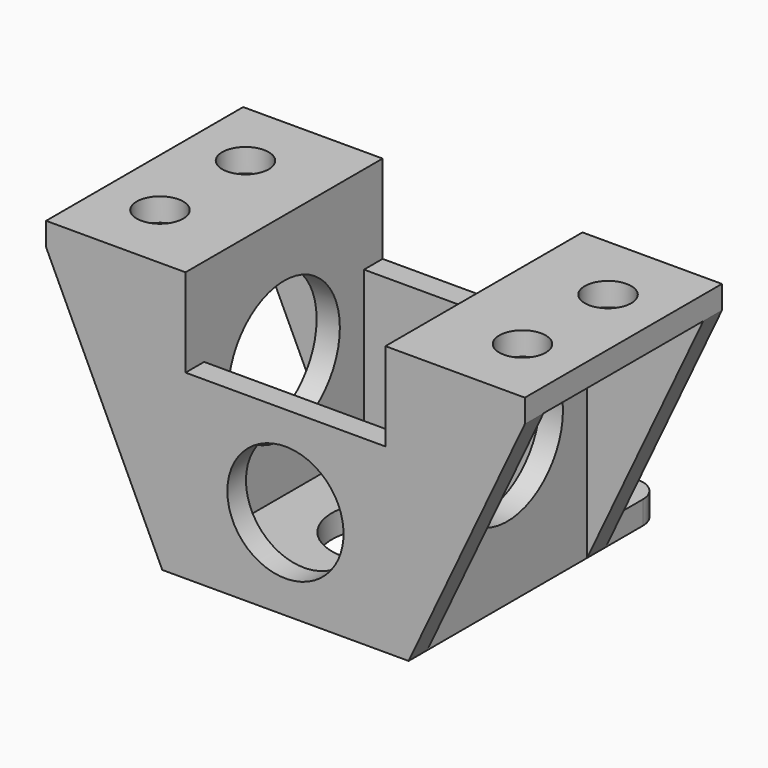
from build123d import *

# Parameters (mm, degrees)
F0_W      = 53
F0_H      = 53
F1_DEPTH  = 10
F2_W      = 43
F2_H      = 43
F3_DEPTH  = 5
F4_R      = 1.7
F5_DEPTH  = 25
F6_R      = 11.2
F7_DEPTH  = 25
F9_DEPTH  = 48
F10_DEPTH = 29
F11_R     = 15
F12_DEPTH = 53.001
F13_R     = 12.5
F14_DEPTH = 53.001
F15_W     = 5
F15_H     = 58
F16_DEPTH = 25
F17_SIZE2 = 53
F17_SIZE  = 25
F18_W     = 43
F18_H     = 5
F19_DEPTH = 25
F20_R     = 5
F21_DEPTH = 25
F22_W     = 15
F22_H     = 5
F23_DEPTH = 15
F24_R     = 5
F25_R     = 4
F26_DEPTH = 25


# Not quite as in the source:
# - a pattern or mirror of a feature is missing from the dataset's text; its kind, count and spacing are read off the source's solid


with BuildPart() as f1:
    # F0 (on Top) → F1 (new body)
    with BuildSketch(Plane.XY):
        Rectangle(F0_W, F0_H)
    extrude(amount=F1_DEPTH)

    # F2 (on face) → F3 (cut)
    with BuildSketch(Plane.XY.offset(10)):
        Rectangle(F2_W, F2_H)
    extrude(amount=-F3_DEPTH, mode=Mode.SUBTRACT)

    # F4 (on face) → F5 (cut)
    with BuildSketch(Plane(origin=(0, 0, 0), x_dir=(1, 0, 0), z_dir=(0, 0, -1))):
        with Locations((-16.5182938799, 16.5182938799)):
            Circle(F4_R)
        with Locations((16.0086180547, 16.5182938799)):
            Circle(F4_R)
        with Locations((16.0086180547, -16.0086180547)):
            Circle(F4_R)
        with Locations((-16.5182938799, -16.0086180547)):
            Circle(F4_R)
    extrude(amount=-F5_DEPTH, mode=Mode.SUBTRACT)

    # F6 (on face) → F7 (cut)
    with BuildSketch(Plane(origin=(0, 0, 0), x_dir=(1, 0, 0), z_dir=(0, 0, -1))):
        Circle(F6_R)
    extrude(amount=-F7_DEPTH, mode=Mode.SUBTRACT)

    # F8 (on face) → F9 (join)
    with BuildSketch(Plane.XY.offset(10)):
        Polygon((-21.5, -21.5), (-21.5, 21.5), (-21.5, 26.5), (-26.5, 26.5), (-26.5, -26.5), (-21.5, -26.5), align=None)
        Polygon((21.5, 26.5), (21.5, 21.5), (21.5, -21.5), (21.5, -26.5), (26.5, -26.5), (26.5, 26.5), align=None)
    extrude(amount=F9_DEPTH)

    # F10 (add): faces of the model
    f10_faces = [f1.faces().sort_by_distance(p)[0] for p in [
        (0, 24, 10),
        (0, -24, 10),
    ]]
    extrude(f10_faces, amount=F10_DEPTH)

    # F11 (on face) → F12 (cut, through all)
    with BuildSketch(Plane.YZ.offset(26.5)):
        with Locations((0, 30.6356716901)):
            Circle(F11_R)
    extrude(amount=-F12_DEPTH, mode=Mode.SUBTRACT)

    # F13 (on face) → F14 (cut, through all)
    with BuildSketch(Plane(origin=(0, 26.5, 0), x_dir=(-1, 0, 0), z_dir=(0, 1, 0))):
        with Locations((0, 19.5)):
            Circle(F13_R)
    extrude(amount=-F14_DEPTH, mode=Mode.SUBTRACT)

    # F15 (on face) → F16 (join)
    with BuildSketch(Plane(origin=(-26.5, 0, 0), x_dir=(0, -1, 0), z_dir=(-1, 0, 0))):
        with Locations((-24, 29)):
            Rectangle(F15_W, F15_H)
        with Locations((24, 29)):
            Rectangle(F15_W, F15_H)
    f16 = extrude(amount=F16_DEPTH)

    # F16_copies: F16 across plane
    add(f16.mirror(Plane(origin=(0, 0, 0), x_dir=(0, 0, 1), z_dir=(1, 0, 0))))

    # F17
    f17_edges = [f1.edges().sort_by_distance(p)[0] for p in [
        (-51.5, 24, 0),
        (-51.5, -24, 0),
        (51.5, 24, 0),
        (51.5, -24, 0),
    ]]
    f17_side = f1.faces().sort_by_distance((25.341639, 0, 0))[0]
    chamfer(f17_edges, length=F17_SIZE, length2=F17_SIZE2, reference=f17_side)

    # F18 (on face) → F19 (join)
    with BuildSketch(Plane(origin=(-26.5, 0, 0), x_dir=(0, -1, 0), z_dir=(-1, 0, 0))):
        with Locations((0, 55.5)):
            Rectangle(F18_W, F18_H)
    f19 = extrude(amount=F19_DEPTH)

    # F19_copies: F19 across plane
    add(f19.mirror(Plane(origin=(0, 0, 0), x_dir=(0, 0, 1), z_dir=(1, 0, 0))))

    # F20 (on face) → F21 (cut)
    with BuildSketch(Plane(origin=(0, 0, 53), x_dir=(1, 0, 0), z_dir=(0, 0, -1))):
        with Locations((-39, 11.5)):
            Circle(F20_R)
        with Locations((-39, -11.5)):
            Circle(F20_R)
    f21 = extrude(amount=-F21_DEPTH, mode=Mode.SUBTRACT)

    # F21_copies: F21 across plane
    add(f21.mirror(Plane(origin=(0, 0, 0), x_dir=(0, 0, 1), z_dir=(1, 0, 0))), mode=Mode.SUBTRACT)

    # F22 (on face) → F23 (join)
    with BuildSketch(Plane(origin=(0, 26.5, 0), x_dir=(-1, 0, 0), z_dir=(0, 1, 0))):
        with Locations((-19, 2.5)):
            Rectangle(F22_W, F22_H)
    f23 = extrude(amount=F23_DEPTH)

    # F23_copies: F23 across plane
    add(f23.mirror(Plane(origin=(0, 0, 0), x_dir=(0, 0, -1), z_dir=(-1, 0, 0))))

    # F24
    f24_edges = [f1.edges().sort_by_distance(p)[0] for p in [
        (11.5, 41.5, 2.5),
        (26.5, 41.5, 2.5),
        (-11.5, 41.5, 2.5),
        (-26.5, 41.5, 2.5),
    ]]
    fillet(f24_edges, radius=F24_R)

    # F25 (on face) → F26 (cut)
    with BuildSketch(Plane(origin=(0, 0, 0), x_dir=(1, 0, 0), z_dir=(0, 0, -1))):
        with Locations((19, -35.5)):
            Circle(F25_R)
    f26 = extrude(amount=-F26_DEPTH, mode=Mode.SUBTRACT)

    # F26_copies: F26 across plane
    add(f26.mirror(Plane(origin=(0, 0, 0), x_dir=(0, 0, -1), z_dir=(-1, 0, 0))), mode=Mode.SUBTRACT)


solid = f1.part
